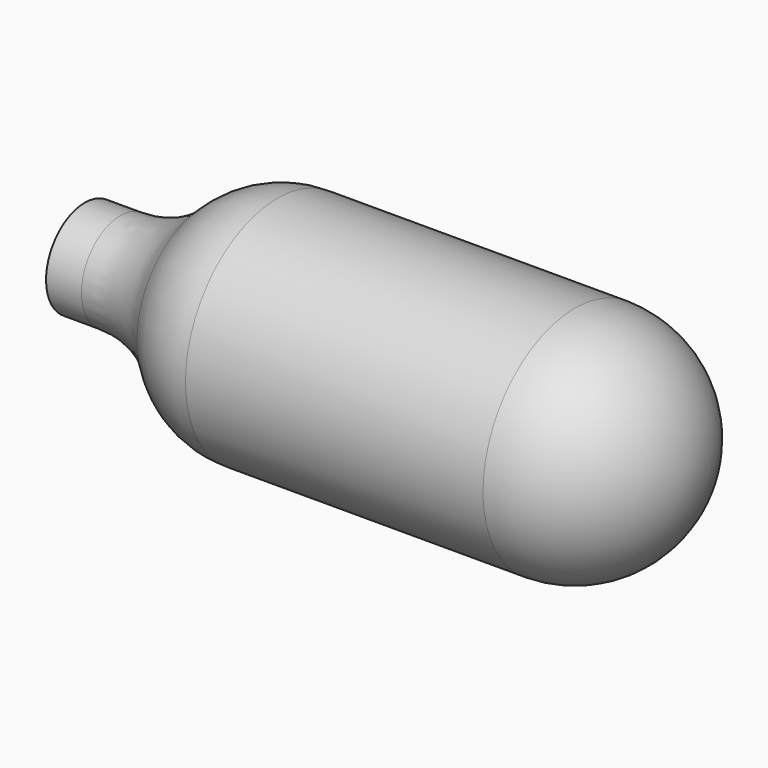
from build123d import *

# Parameters (mm, degrees)
F2_R = 9.5
F4_R = 9.6520512263


# Not quite as in the source:
# - a fillet or chamfer that OpenCascade refuses, or shapes differently, is made with other operations: its cross-section is extruded or revolved along the edge and cut away or added


with BuildPart() as f1:
    # F0 (on Front) → F1 (revolve)
    with BuildSketch(Plane.XZ):
        Polygon((0, 4), (0, 0), (50, 0), (50, 9.5), (8, 9.5), (8, 4), align=None)
    revolve(axis=Axis((25, 0, 0), (-1, 0, 0)))

    # F2
    f2_edges = [f1.edges().sort_by_distance(p)[0] for p in [
        (50, 0, -9.5),
    ]]
    fillet(f2_edges, radius=F2_R)

    # F3: fillet of radius 8.4497474683 on 1 edges, made by hand

    # F3_s1 → F3_t2 (revolve, cut)
    with BuildSketch(Plane.XZ):
        with BuildLine():
            ThreePointArc((15.9181577498, 9.5), (11.0977007655, 7.990095955), (8, 4))
            Line((8, 4), (8, 9.5))
            Line((8, 9.5), (15.9181577498, 9.5))
        make_face()
    revolve(axis=Axis((8, 0, 0), (-1, 0, 0)), mode=Mode.SUBTRACT)

    # F4
    f4_edges = [f1.edges().sort_by_distance(p)[0] for p in [
        (8, 0, -4),
    ]]
    fillet(f4_edges, radius=F4_R)


solid = f1.part
